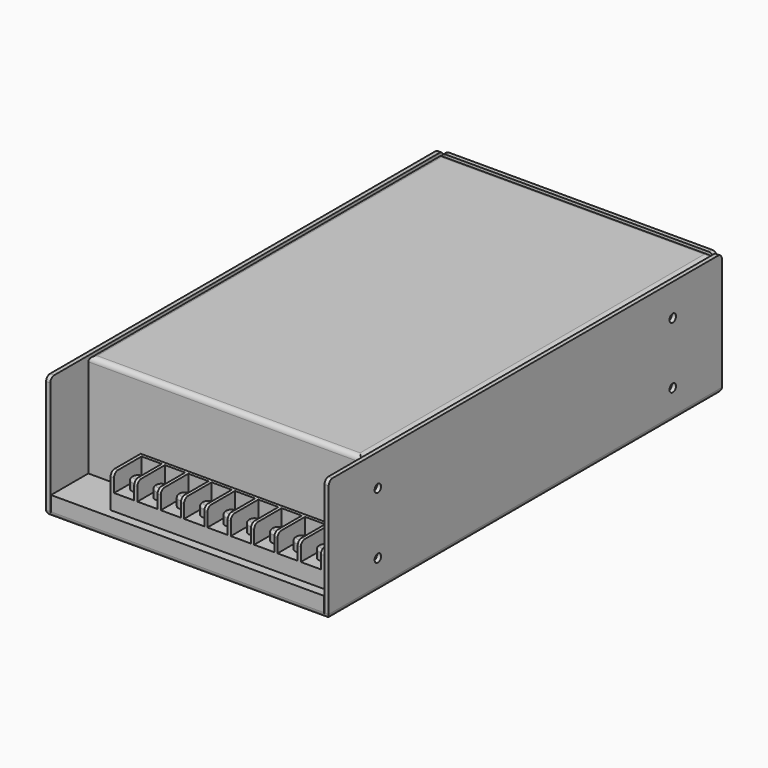
from build123d import *

# Parameters (mm, degrees)
F0_W             = 57.5
F0_H             = 50
F1_DEPTH         = 100
F2_W             = 55.8
F2_H             = 19
F3_DEPTH         = 42
F4_W             = 0.3
F4_H             = 19
F5_DEPTH         = 48.3
F8_W             = 87
F8_H             = 15.3
F9_DEPTH         = 14
F10_W            = 8.2
F10_H            = 14
F11_DEPTH        = 7.4
F12_F1_R         = 2
F12_F2_R         = 2
F12_F3_R         = 2
F12_F4_R         = 2
F12_F5_R         = 2
F12_F6_R         = 2
F12_F7_R         = 2
F12_F8_R         = 2
F12_F9_R         = 2
F12_F10_R        = 2
F12_2_T1_DEPTH   = 189
F12_2_T3_DEPTH   = 11.7
F12_2_T5_DEPTH   = 125
F12_2_T7_DEPTH   = 11.7
F12_2_T9_DEPTH   = 6.7
F12_2_T11_DEPTH  = 11.7
F12_2_T13_DEPTH  = 210
F12_2_T18_DEPTH  = 116
F12_2_T23_DEPTH  = 116
F12_2_T28_DEPTH  = 11.7
F13_R            = 2.5
F14_DEPTH        = 4
F15_R            = 1
F19_D            = 3.3
F19_DEPTH        = 5
F19_TIP          = 0.9914200214
F19_ON_F18_D     = 3.3
F19_ON_F18_DEPTH = 5
F19_ON_F18_TIP   = 0.9914200214
F19_ON_F17_D     = 3.3
F19_ON_F17_DEPTH = 5
F19_ON_F17_TIP   = 0.9914200214


# Not quite as in the source:
# - a fillet or chamfer that OpenCascade refuses, or shapes differently, is made with other operations: its cross-section is extruded or revolved along the edge and cut away or added
# - a feature of the source that left no trace in its solid (it failed there, or was rolled back) is left out


with BuildPart() as f1:
    # F0 (on Front) → F1 (new body, symmetric)
    with BuildSketch(Plane.XZ):
        with Locations((-28.75, 0)):
            Rectangle(F0_W, F0_H)
    extrude(amount=F1_DEPTH, both=True)

    # F2 (on face) → F3 (cut)
    with BuildSketch(Plane.XY.offset(25)):
        with Locations((-27.9, -90.5)):
            Rectangle(F2_W, F2_H)
    extrude(amount=-F3_DEPTH, mode=Mode.SUBTRACT)

    # F4 (on face) → F5 (cut)
    with BuildSketch(Plane.XY.offset(25)):
        Polygon((-55.8, 100), (-55.8, -81), (-55.5, -81), (-55.5, 98), (0, 98), (0, 98.3), (-55.5, 98.3), (-55.5, 100), align=None)
        with Locations((-55.65, -90.5)):
            Rectangle(F4_W, F4_H)
    extrude(amount=-F5_DEPTH, mode=Mode.SUBTRACT)

    # F7: F1 across plane


with BuildPart() as f1_1:
    add(f1.part)
    add(f1.part.mirror(Plane.YZ))

    # F12#2: fillet of radius 2 on 14 edges, made by hand

    # F12_2_s2 → F12_2_t1 (cut)
    with BuildSketch(Plane.XZ.offset(-103)):
        with BuildLine():
            ThreePointArc((53.5, 25), (54.9142135624, 24.4142135624), (55.5, 23))
            Line((55.5, 23), (55.5, 25))
            Line((55.5, 25), (53.5, 25))
        make_face()
        with BuildLine():
            ThreePointArc((-53.5, 25), (-54.9142135624, 24.4142135624), (-55.5, 23))
            Line((-55.5, 23), (-55.5, 25))
            Line((-55.5, 25), (-53.5, 25))
        make_face()
    extrude(amount=F12_2_T1_DEPTH, mode=Mode.SUBTRACT)

    # F12_2_s4 → F12_2_t3 (cut)
    with BuildSketch(Plane.YZ.offset(-62.5)):
        with BuildLine():
            ThreePointArc((-100, 23), (-99.4142135624, 24.4142135624), (-98, 25))
            Line((-98, 25), (-100, 25))
            Line((-100, 25), (-100, 23))
        make_face()
    extrude(amount=F12_2_T3_DEPTH, mode=Mode.SUBTRACT)

    # F12_2_s6 → F12_2_t5 (cut)
    with BuildSketch(Plane.YZ.offset(-62.5)):
        with BuildLine():
            ThreePointArc((-100, -23), (-99.4142135624, -24.4142135624), (-98, -25))
            Line((-98, -25), (-100, -25))
            Line((-100, -25), (-100, -23))
        make_face()
        with BuildLine():
            ThreePointArc((100, -23), (99.4142135624, -24.4142135624), (98, -25))
            Line((98, -25), (100, -25))
            Line((100, -25), (100, -23))
        make_face()
    extrude(amount=F12_2_T5_DEPTH, mode=Mode.SUBTRACT)

    # F12_2_s8 → F12_2_t7 (cut)
    with BuildSketch(Plane.YZ.offset(50.8)):
        with BuildLine():
            ThreePointArc((-100, 23), (-99.4142135624, 24.4142135624), (-98, 25))
            Line((-98, 25), (-100, 25))
            Line((-100, 25), (-100, 23))
        make_face()
    extrude(amount=F12_2_T7_DEPTH, mode=Mode.SUBTRACT)

    # F12_2_s10 → F12_2_t9 (cut)
    with BuildSketch(Plane.YZ.offset(-62.5)):
        with BuildLine():
            ThreePointArc((100, 23), (99.4142135624, 24.4142135624), (98, 25))
            Line((98, 25), (100, 25))
            Line((100, 25), (100, 23))
        make_face()
    extrude(amount=F12_2_T9_DEPTH, mode=Mode.SUBTRACT)

    # F12_2_s12 → F12_2_t11 (cut)
    with BuildSketch(Plane.XZ.offset(-105)):
        with BuildLine():
            ThreePointArc((-55.5, 23), (-54.9142135624, 24.4142135624), (-53.5, 25))
            Line((-53.5, 25), (-55.5, 25))
            Line((-55.5, 25), (-55.5, 23))
        make_face()
        with BuildLine():
            ThreePointArc((53.5, 25), (54.9142135624, 24.4142135624), (55.5, 23))
            Line((55.5, 23), (55.5, 25))
            Line((55.5, 25), (53.5, 25))
        make_face()
    extrude(amount=F12_2_T11_DEPTH, mode=Mode.SUBTRACT)

    # F12_2_s14 → F12_2_t13 (cut)
    with BuildSketch(Plane.XZ.offset(-105)):
        with BuildLine():
            ThreePointArc((57.5, -23), (56.9142135624, -24.4142135624), (55.5, -25))
            Line((55.5, -25), (57.5, -25))
            Line((57.5, -25), (57.5, -23))
        make_face()
        with BuildLine():
            ThreePointArc((-55.5, -25), (-56.9142135624, -24.4142135624), (-57.5, -23))
            Line((-57.5, -23), (-57.5, -25))
            Line((-57.5, -25), (-55.5, -25))
        make_face()
    extrude(amount=F12_2_T13_DEPTH, mode=Mode.SUBTRACT)


with BuildPart() as f9:
    # F8 (on face) → F9 (new body)
    with BuildSketch(Plane.XY.offset(-17)):
        with Locations((9.3, -88.65)):
            Rectangle(F8_W, F8_H)
    extrude(amount=F9_DEPTH)

    # F10 (on face) → F11 (cut)
    with BuildSketch(Plane.XY.offset(-3)):
        with Locations((-28.7, -89.3)):
            Rectangle(F10_W, F10_H)
        with Locations((-19.2, -89.3)):
            Rectangle(F10_W, F10_H)
        with Locations((-9.7, -89.3)):
            Rectangle(F10_W, F10_H)
        with Locations((-0.2, -89.3)):
            Rectangle(F10_W, F10_H)
        with Locations((9.3, -89.3)):
            Rectangle(F10_W, F10_H)
        with Locations((18.8, -89.3)):
            Rectangle(F10_W, F10_H)
        with Locations((28.3, -89.3)):
            Rectangle(F10_W, F10_H)
        with Locations((37.8, -89.3)):
            Rectangle(F10_W, F10_H)
        with Locations((47.3, -89.3)):
            Rectangle(F10_W, F10_H)
    extrude(amount=-F11_DEPTH, mode=Mode.SUBTRACT)

    # F12: fillet of radius 2 on 10 edges, made by hand

    # F12_f1
    f12_f1_edges = [f9.edges().sort_by_distance(p)[0] for p in [
        (52.1, -96.3, -3),
    ]]
    fillet(f12_f1_edges, radius=F12_F1_R)

    # F12_f2
    f12_f2_edges = [f9.edges().sort_by_distance(p)[0] for p in [
        (42.55, -96.3, -3),
    ]]
    fillet(f12_f2_edges, radius=F12_F2_R)

    # F12_f3
    f12_f3_edges = [f9.edges().sort_by_distance(p)[0] for p in [
        (33.05, -96.3, -3),
    ]]
    fillet(f12_f3_edges, radius=F12_F3_R)

    # F12_f4
    f12_f4_edges = [f9.edges().sort_by_distance(p)[0] for p in [
        (23.55, -96.3, -3),
    ]]
    fillet(f12_f4_edges, radius=F12_F4_R)

    # F12_f5
    f12_f5_edges = [f9.edges().sort_by_distance(p)[0] for p in [
        (14.05, -96.3, -3),
    ]]
    fillet(f12_f5_edges, radius=F12_F5_R)

    # F12_f6
    f12_f6_edges = [f9.edges().sort_by_distance(p)[0] for p in [
        (4.55, -96.3, -3),
    ]]
    fillet(f12_f6_edges, radius=F12_F6_R)

    # F12_f7
    f12_f7_edges = [f9.edges().sort_by_distance(p)[0] for p in [
        (-4.95, -96.3, -3),
    ]]
    fillet(f12_f7_edges, radius=F12_F7_R)

    # F12_f8
    f12_f8_edges = [f9.edges().sort_by_distance(p)[0] for p in [
        (-14.45, -96.3, -3),
    ]]
    fillet(f12_f8_edges, radius=F12_F8_R)

    # F12_f9
    f12_f9_edges = [f9.edges().sort_by_distance(p)[0] for p in [
        (-23.95, -96.3, -3),
    ]]
    fillet(f12_f9_edges, radius=F12_F9_R)

    # F12_f10
    f12_f10_edges = [f9.edges().sort_by_distance(p)[0] for p in [
        (-33.5, -96.3, -3),
    ]]
    fillet(f12_f10_edges, radius=F12_F10_R)

    # F13 (on face) → F14 (join)
    with BuildSketch(Plane.XY.offset(-10.4)):
        with Locations((-28.7, -89.3)):
            Circle(F13_R)
        with Locations((-19.2, -89.3)):
            Circle(F13_R)
        with Locations((-9.7, -89.3)):
            Circle(F13_R)
        with Locations((-0.2, -89.3)):
            Circle(F13_R)
        with Locations((9.3, -89.3)):
            Circle(F13_R)
        with Locations((18.8, -89.3)):
            Circle(F13_R)
        with Locations((28.3, -89.3)):
            Circle(F13_R)
        with Locations((37.8, -89.3)):
            Circle(F13_R)
        with Locations((47.3, -89.3)):
            Circle(F13_R)
    extrude(amount=F14_DEPTH)

    # F15
    f15_edges = [f9.edges().sort_by_distance(p)[0] for p in [
        (-31.2, -89.3, -6.4),
        (-21.7, -89.3, -6.4),
        (-12.2, -89.3, -6.4),
        (-2.7, -89.3, -6.4),
        (6.8, -89.3, -6.4),
        (16.3, -89.3, -6.4),
        (25.8, -89.3, -6.4),
        (35.3, -89.3, -6.4),
        (44.8, -89.3, -6.4),
    ]]
    fillet(f15_edges, radius=F15_R)


with BuildPart() as f12_2_tool16:
    # F12_2_s17 → F12_2_t18 (new body)
    with BuildSketch(Plane.YZ.offset(-60.5)):
        with BuildLine():
            ThreePointArc((-79, 25), (-80.4142135624, 24.4142135624), (-81, 23))
            Line((-81, 23), (-81, 25))
            Line((-81, 25), (-79, 25))
        make_face()
    extrude(amount=F12_2_T18_DEPTH)

    split(bisect_by=Plane.YZ.offset(-55.8), keep=Keep.TOP)


with BuildPart() as f1_2:
    add(f1_1.part)

    # F12_2_t15: cut F12_2_tool16
    add(f12_2_tool16.part, mode=Mode.SUBTRACT)


with BuildPart() as f12_2_tool21:
    # F12_2_s22 → F12_2_t23 (new body)
    with BuildSketch(Plane.YZ.offset(55.5)):
        with BuildLine():
            ThreePointArc((96, 25), (97.4142135624, 24.4142135624), (98, 23))
            Line((98, 23), (98, 25))
            Line((98, 25), (96, 25))
        make_face()
    extrude(amount=-F12_2_T23_DEPTH)

    split(bisect_by=Plane.YZ.offset(-55.8), keep=Keep.TOP)


with BuildPart() as f1_3:
    add(f1_2.part)

    # F12_2_t20: cut F12_2_tool21
    add(f12_2_tool21.part, mode=Mode.SUBTRACT)


with BuildPart() as f12_2_tool26:
    # F12_2_s27 → F12_2_t28 (new body)
    with BuildSketch(Plane.YZ.offset(50.8)):
        with BuildLine():
            ThreePointArc((100, 23), (99.4142135624, 24.4142135624), (98, 25))
            Line((98, 25), (100, 25))
            Line((100, 25), (100, 23))
        make_face()
    extrude(amount=F12_2_T28_DEPTH)

    split(bisect_by=Plane.YZ.offset(55.5), keep=Keep.TOP)


with BuildPart() as f1_4:
    add(f1_3.part)

    # F12_2_t25: cut F12_2_tool26
    add(f12_2_tool26.part, mode=Mode.SUBTRACT)

    # F19
    with Locations(Plane(origin=(-57.5, 0, 0), x_dir=(0, -1, 0), z_dir=(-1, 0, 0))):
        with Locations((-75, -13), (75, -13)):
            Hole(F19_D / 2, depth=F19_DEPTH)
            with Locations((0, 0, -(F19_DEPTH + F19_TIP / 2))):  # 118° drill point
                Cone(0, F19_D / 2, F19_TIP, mode=Mode.SUBTRACT)

    # F19 on F18
    with Locations(Plane(origin=(0, 0, -25), x_dir=(1, 0, 0), z_dir=(0, 0, -1))):
        with Locations((-25, -75), (-25, 75), (25, -75), (25, 75)):
            Hole(F19_ON_F18_D / 2, depth=F19_ON_F18_DEPTH)
            with Locations((0, 0, -(F19_ON_F18_DEPTH + F19_ON_F18_TIP / 2))):  # 118° drill point
                Cone(0, F19_ON_F18_D / 2, F19_ON_F18_TIP, mode=Mode.SUBTRACT)

    # F19 on F17
    with Locations(Plane.YZ.offset(57.5)):
        with Locations((-75, -13), (-75, 12), (75, 12), (75, -13)):
            Hole(F19_ON_F17_D / 2, depth=F19_ON_F17_DEPTH)
            with Locations((0, 0, -(F19_ON_F17_DEPTH + F19_ON_F17_TIP / 2))):  # 118° drill point
                Cone(0, F19_ON_F17_D / 2, F19_ON_F17_TIP, mode=Mode.SUBTRACT)


solid = Compound([f9.part, f1_4.part])
